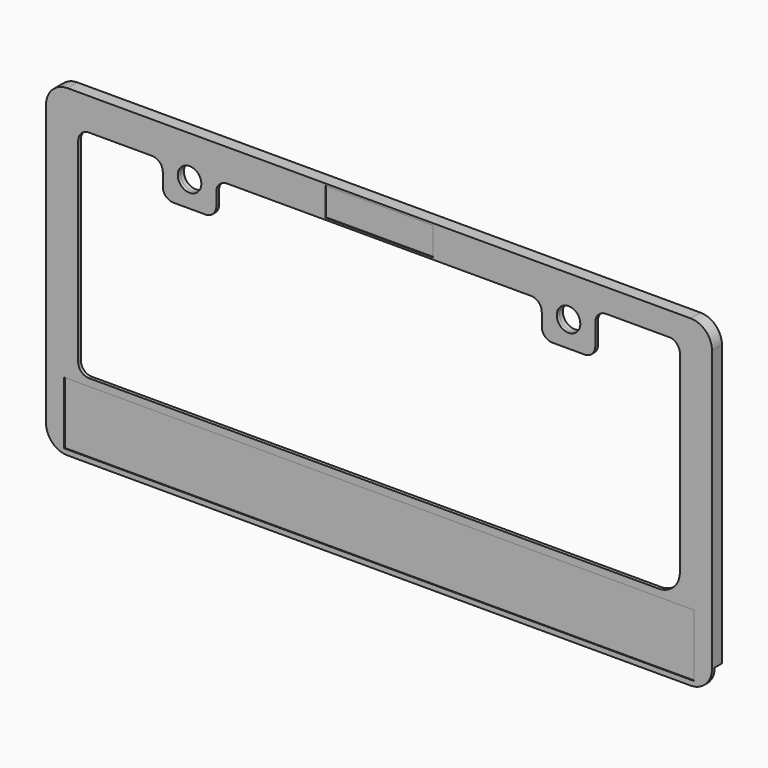
from build123d import *
from build123d import SkipClean  # not in build123d's __all__

# Parameters (mm, degrees)
F1_DEPTH  = 1.6
F2_W      = 25
F2_H      = 16
F3_DEPTH  = 1.6
F5_DEPTH  = 25
F6_R      = 5
F8_R      = 5.5
F9_DEPTH  = 25
F12_R     = 8.5
F12_R_2   = 5.5
F13_DEPTH = 2
F15_DEPTH = 4.2
F17_DEPTH = 1.6
F19_W     = 294.2
F19_H     = 29.2
F19_W_2   = 50.2
F19_H_2   = 13.2
F20_DEPTH = 0.4


# Not quite as in the source:
# - two fillets or chamfers of one size are made in one step
# - after a boolean that leaves OpenCascade's solid faulty, fix() repairs it


with BuildPart() as f1:
    # F0 (on Front) → F1 (new body)
    with BuildSketch(Plane.XZ):
        with BuildLine():
            ThreePointArc((155.5, 65.5), (152.5710678119, 72.5710678119), (145.5, 75.5))
            Line((145.5, 75.5), (-145.5, 75.5))
            ThreePointArc((-145.5, 75.5), (-152.5710678119, 72.5710678119), (-155.5, 65.5))
            Line((-155.5, 65.5), (-155.5, -65.5))
            ThreePointArc((-155.5, -65.5), (-152.5710678119, -72.5710678119), (-145.5, -75.5))
            Line((-145.5, -75.5), (145.5, -75.5))
            ThreePointArc((145.5, -75.5), (152.5710678119, -72.5710678119), (155.5, -65.5))
            Line((155.5, -65.5), (155.5, 65.5))
        make_face()
        with BuildLine():
            Line((-135.5, 60.5), (135.5, 60.5))
            ThreePointArc((135.5, 60.5), (139.0355339059, 59.0355339059), (140.5, 55.5))
            Line((140.5, 55.5), (140.5, -30.5))
            ThreePointArc((140.5, -30.5), (137.5710678119, -37.5710678119), (130.5, -40.5))
            Line((130.5, -40.5), (-135.5, -40.5))
            ThreePointArc((-135.5, -40.5), (-139.0355339059, -39.0355339059), (-140.5, -35.5))
            Line((-140.5, -35.5), (-140.5, 55.5))
            ThreePointArc((-140.5, 55.5), (-139.0355339059, 59.0355339059), (-135.5, 60.5))
        make_face(mode=Mode.SUBTRACT)
    extrude(amount=F1_DEPTH)

    # F2 (on face) → F3 (join, through all)
    with BuildSketch(Plane.XZ.offset(1.6)):
        with Locations((-88.5, 52.5)):
            Rectangle(F2_W, F2_H)
        with Locations((88.5, 52.5)):
            Rectangle(F2_W, F2_H)
    extrude(amount=-F3_DEPTH)

    # F4 (on face) → F5 (cut)
    with BuildSketch(Plane.XZ.offset(1.6)):
        Polygon((101, 64.5), (101, 60.5), (101, 55.5), (140.5, 55.5), (140.5, 64.5), align=None)
    extrude(amount=-F5_DEPTH, mode=Mode.SUBTRACT)

    # F6
    f6_edges = [f1.edges().sort_by_distance(p)[0] for p in [
        (-101, -0.8, 44.5),
        (-101, -0.8, 60.5),
        (-76, -0.8, 44.5),
        (-76, -0.8, 60.5),
        (101, -0.8, 44.5),
        (76, -0.8, 44.5),
        (76, -0.8, 60.5),
        (140.5, -0.8, 64.5),
        (101, -0.8, 64.5),
    ]]
    fillet(f6_edges, radius=F6_R)

    # F8 (on face) → F9 (cut)
    with BuildSketch(Plane.XZ.offset(1.6)):
        with Locations((-88.5, 56.5)):
            Circle(F8_R)
        with Locations((88.5, 56.5)):
            Circle(F8_R)
    extrude(amount=-F9_DEPTH, mode=Mode.SUBTRACT)

    # F12 (on face) → F13 (join)
    with BuildSketch(Plane(origin=(0, 0, 0), x_dir=(-1, 0, 0), z_dir=(0, 1, 0))):
        with Locations((-88.5, 56.5)):
            Circle(F12_R)
        with Locations((-88.5, 56.5)):
            Circle(F12_R_2, mode=Mode.SUBTRACT)
        with Locations((88.5, 56.5)):
            Circle(F12_R)
        with Locations((88.5, 56.5)):
            Circle(F12_R_2, mode=Mode.SUBTRACT)
    with SkipClean():  # cleaning this boolean's faces spoils the solid; the shape is the same uncleaned
        extrude(amount=F13_DEPTH)

    # F14 (on face) → F15 (join)
    with BuildSketch(Plane(origin=(0, 0, 0), x_dir=(-1, 0, 0), z_dir=(0, 1, 0))):
        with BuildLine():
            ThreePointArc((-145.5, 75.5), (-152.5710678119, 72.5710678119), (-155.5, 65.5))
            Line((-155.5, 65.5), (-155.5, -65.5))
            Line((-155.5, -65.5), (-153.5, -65.5))
            Line((-153.5, -65.5), (-153.5, 65.5))
            ThreePointArc((-153.5, 65.5), (-151.1568542495, 71.1568542495), (-145.5, 73.5))
            Line((-145.5, 73.5), (145.5, 73.5))
            ThreePointArc((145.5, 73.5), (151.1568542495, 71.1568542495), (153.5, 65.5))
            Line((153.5, 65.5), (153.5, -65.5))
            Line((153.5, -65.5), (155.5, -65.5))
            Line((155.5, -65.5), (155.5, 65.5))
            ThreePointArc((155.5, 65.5), (152.5710678119, 72.5710678119), (145.5, 75.5))
            Line((145.5, 75.5), (-145.5, 75.5))
        make_face()
    extrude(amount=F15_DEPTH)

    add(f1.part.fix(), mode=Mode.REPLACE)

    # F16 (on face) → F17 (join)
    with BuildSketch(Plane(origin=(0, 4.2, 0), x_dir=(-1, 0, 0), z_dir=(0, 1, 0))):
        Polygon((-153.5, 31), (-153.5, -31), (-146.5, -31), (-146.5, 22.6577248518), align=None)
        Polygon((146.5, -31), (153.5, -31), (153.5, 31), (146.5, 22.6577248518), align=None)
    extrude(amount=-F17_DEPTH)

    # F19 (on face) → F20 (cut)
    with BuildSketch(Plane.XZ.offset(1.6)):
        with Locations((0, -58.5)):
            Rectangle(F19_W, F19_H)
        with Locations((0, 68)):
            Rectangle(F19_W_2, F19_H_2)
    extrude(amount=-F20_DEPTH, mode=Mode.SUBTRACT)


solid = f1.part
